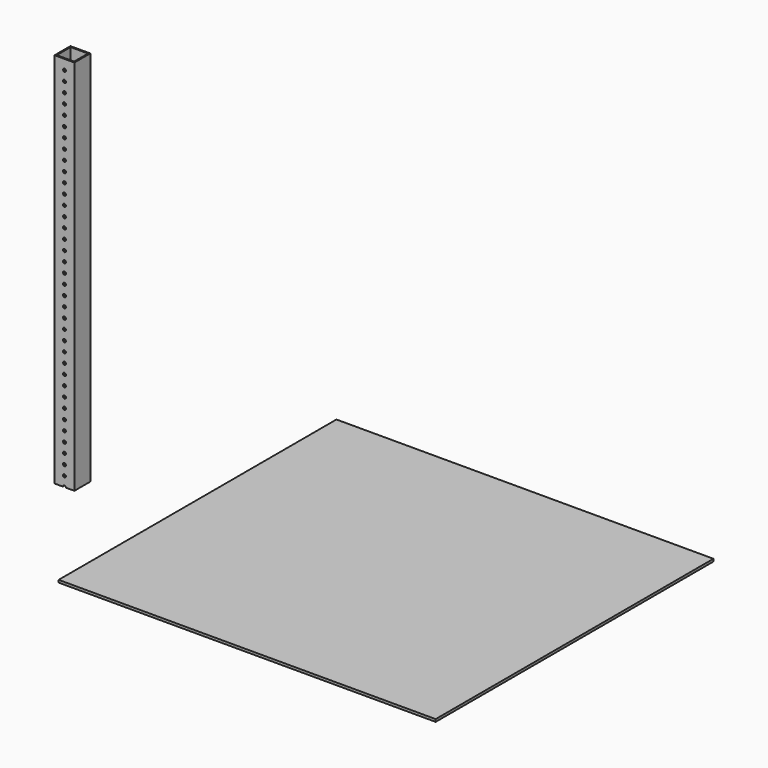
from build123d import *

# Parameters (mm, degrees)
F0_W     = 25.4
F0_H     = 25.4
F0_W_2   = 22.225
F0_H_2   = 22.225
F1_DEPTH = 482.6
F2_R     = 1.905
F3_DEPTH = 25.401
F4_W     = 482.6
F4_H     = 444.5
F5_DEPTH = 3.175


# Not quite as in the source:
# - a length typed as a fraction of an inch, garbled in the dataset ("3 / 203.2 mm" for 3/8 in), is restored


with BuildPart() as f1:
    # F0 (on Top) → F1 (new body)
    with BuildSketch(Plane.XY):
        with Locations((-53.6350669761, 38.1377951519)):
            Rectangle(F0_W, F0_H)
        with Locations((-53.6350669761, 38.1377951519)):
            Rectangle(F0_W_2, F0_H_2, mode=Mode.SUBTRACT)
    extrude(amount=F1_DEPTH)

    # F2 (on face) → F3 (cut, through all)
    with BuildSketch(Plane.XZ.offset(-25.4377951519)):
        with Locations((-53.6350669761, 469.9)):
            Circle(F2_R)
        with Locations((-53.6350669761, 457.2)):
            Circle(F2_R)
        with Locations((-53.6350669761, 444.5)):
            Circle(F2_R)
        with Locations((-53.6350669761, 431.8)):
            Circle(F2_R)
        with Locations((-53.6350669761, 419.1)):
            Circle(F2_R)
        with Locations((-53.6350669761, 406.4)):
            Circle(F2_R)
        with Locations((-53.6350669761, 393.7)):
            Circle(F2_R)
        with Locations((-53.6350669761, 381)):
            Circle(F2_R)
        with Locations((-53.6350669761, 368.3)):
            Circle(F2_R)
        with Locations((-53.6350669761, 355.6)):
            Circle(F2_R)
        with Locations((-53.6350669761, 342.9)):
            Circle(F2_R)
        with Locations((-53.6350669761, 330.2)):
            Circle(F2_R)
        with Locations((-53.6350669761, 317.5)):
            Circle(F2_R)
        with Locations((-53.6350669761, 304.8)):
            Circle(F2_R)
        with Locations((-53.6350669761, 292.1)):
            Circle(F2_R)
        with Locations((-53.6350669761, 279.4)):
            Circle(F2_R)
        with Locations((-53.6350669761, 266.7)):
            Circle(F2_R)
        with Locations((-53.6350669761, 254)):
            Circle(F2_R)
        with Locations((-53.6350669761, 241.3)):
            Circle(F2_R)
        with Locations((-53.6350669761, 228.6)):
            Circle(F2_R)
        with Locations((-53.6350669761, 215.9)):
            Circle(F2_R)
        with Locations((-53.6350669761, 203.2)):
            Circle(F2_R)
        with Locations((-53.6350669761, 190.5)):
            Circle(F2_R)
        with Locations((-53.6350669761, 177.8)):
            Circle(F2_R)
        with Locations((-53.6350669761, 165.1)):
            Circle(F2_R)
        with Locations((-53.6350669761, 152.4)):
            Circle(F2_R)
        with Locations((-53.6350669761, 139.7)):
            Circle(F2_R)
        with Locations((-53.6350669761, 127)):
            Circle(F2_R)
        with Locations((-53.6350669761, 114.3)):
            Circle(F2_R)
        with Locations((-53.6350669761, 101.6)):
            Circle(F2_R)
        with Locations((-53.6350669761, 88.9)):
            Circle(F2_R)
        with Locations((-53.6350669761, 76.2)):
            Circle(F2_R)
        with Locations((-53.6350669761, 63.5)):
            Circle(F2_R)
        with Locations((-53.6350669761, 50.8)):
            Circle(F2_R)
        with Locations((-53.6350669761, 38.1)):
            Circle(F2_R)
        with Locations((-53.6350669761, 25.4)):
            Circle(F2_R)
        with Locations((-53.6350669761, 12.7)):
            Circle(F2_R)
        with Locations((-53.6350669761, 0)):
            Circle(F2_R)
        with Locations((-53.6350669761, -12.7)):
            Circle(F2_R)
        with Locations((-53.6350669761, -25.4)):
            Circle(F2_R)
    extrude(amount=-F3_DEPTH, mode=Mode.SUBTRACT)


with BuildPart() as f5:
    # F4 (on Top) → F5 (new body)
    with BuildSketch(Plane.XY):
        with Locations((312.2163708924, 82.6781136751)):
            Rectangle(F4_W, F4_H)
    extrude(amount=F5_DEPTH)


solid = Compound([f1.part, f5.part])
